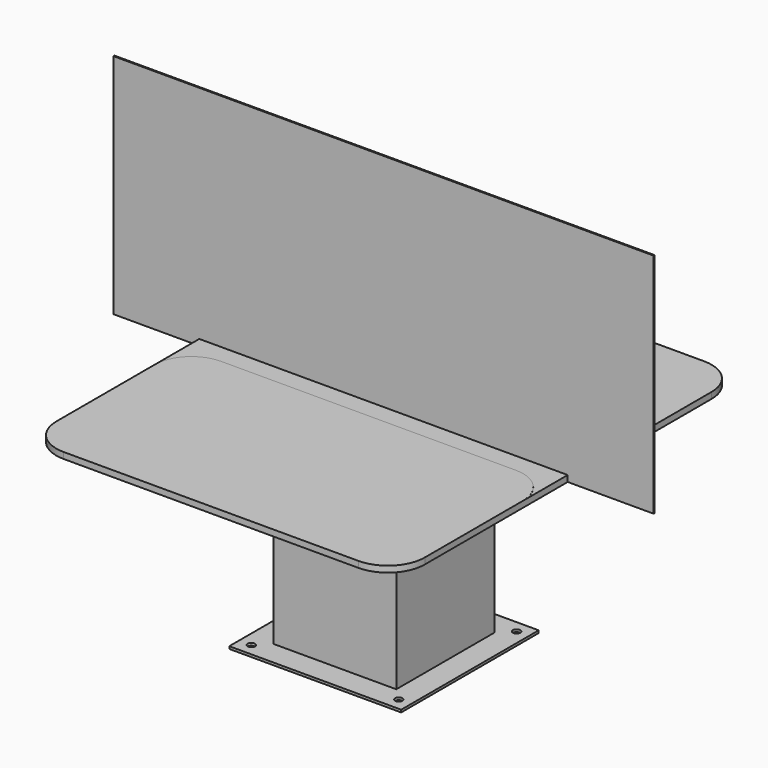
from build123d import *

# Parameters (mm, degrees)
F0_R      = 1250
F1_DEPTH  = 25
F3_DEPTH  = 0.1
F4_W      = 500
F4_H      = 500
F4_W_2    = 490
F4_H_2    = 490
F5_DEPTH  = 800
F6_W      = 2200
F6_H      = 5
F7_DEPTH  = 900
F8_W      = 500
F8_H      = 500
F9_DEPTH  = 5
F10_W     = 700
F10_H     = 700
F10_R     = 15
F11_DEPTH = 10
F13_DEPTH = 30
F15_DEPTH = 30
F16_W     = 490
F16_H     = 490
F17_DEPTH = 25
F18_R     = 350
F20_DEPTH = 25
F21_W     = 350
F21_H     = 25
F22_DEPTH = 5


# Not quite as in the source:
# - a feature names something its author has since deleted; it is built from what else it names


with BuildPart() as f1:
    # F0 (on Top) → F1 (new body)
    with BuildSketch(Plane.XY):
        Circle(F0_R)
    extrude(amount=F1_DEPTH)

    # F2 (on face) → F3 (join)
    with BuildSketch(Plane.XY.offset(25)):
        with BuildLine():
            Line((-600, 80), (600, 80))
            ThreePointArc((600, 80), (706.066017178, 123.933982822), (750, 230))
            Line((750, 230), (750, 730))
            ThreePointArc((750, 730), (706.066017178, 836.066017178), (600, 880))
            Line((600, 880), (-600, 880))
            ThreePointArc((-600, 880), (-706.066017178, 836.066017178), (-750, 730))
            Line((-750, 730), (-750, 230))
            ThreePointArc((-750, 230), (-706.066017178, 123.933982822), (-600, 80))
        make_face()
        with BuildLine():
            ThreePointArc((-600, -80), (-706.066017178, -123.933982822), (-750, -230))
            Line((-750, -230), (-750, -730))
            ThreePointArc((-750, -730), (-706.066017178, -836.066017178), (-600, -880))
            Line((-600, -880), (600, -880))
            ThreePointArc((600, -880), (706.066017178, -836.066017178), (750, -730))
            Line((750, -730), (750, -230))
            ThreePointArc((750, -230), (706.066017178, -123.933982822), (600, -80))
            Line((600, -80), (-600, -80))
        make_face()
    extrude(amount=F3_DEPTH)

    # F12 (on face) → F13 (cut)
    with BuildSketch(Plane.XY.offset(25)):
        with BuildLine():
            ThreePointArc((835.2245207129, -930), (0, -1250), (-835.2245207129, -930))
            Line((-835.2245207129, -930), (-1254.9974999975, -930))
            Line((-1254.9974999975, -930), (-1254.9974999975, -1430))
            Line((-1254.9974999975, -1430), (1245.0025000025, -1430))
            Line((1245.0025000025, -1430), (1245.0025000025, -930))
            Line((1245.0025000025, -930), (835.2245207129, -930))
        make_face()
        with BuildLine():
            Line((-835.2245207129, 930), (835.2245207129, 930))
            ThreePointArc((835.2245207129, 930), (0, 1250), (-835.2245207129, 930))
        make_face()
        with BuildLine():
            Line((835.2245207129, -930), (-835.2245207129, -930))
            ThreePointArc((-835.2245207129, -930), (0, -1250), (835.2245207129, -930))
        make_face()
    extrude(amount=-F13_DEPTH, mode=Mode.SUBTRACT)

    # F14 (on face) → F15 (cut)
    with BuildSketch(Plane.XY.offset(25)):
        Polygon((835.2245207128, 930), (835.2245207128, -930), (1324.2889336484, -826), (1324.2889336484, 930), align=None)
        Polygon((-1324.2889336484, -826), (-835.2245207128, -930), (-835.2245207128, 930), (-1324.2889336484, 930), align=None)
    extrude(amount=-F15_DEPTH, mode=Mode.SUBTRACT)

    # F18
    f18_edges = [f1.edges().sort_by_distance(p)[0] for p in [
        (-835.224521, 930, 12.5),
        (-835.224521, -930, 12.5),
        (835.224521, -930, 12.5),
        (835.224521, 930, 12.5),
    ]]
    fillet(f18_edges, radius=F18_R)

    # F19 (on face) → F20 (cut)
    with BuildSketch(Plane.XY.offset(25)):
        with BuildLine():
            Line((-750, 230), (-750, 730))
            ThreePointArc((-750, 730), (-730.6905446057, 803.6205239771), (-677.7335793245, 858.2867516363))
            Line((-677.7335793245, 858.2867516363), (-665.502084486, 880))
            ThreePointArc((-665.502084486, 880), (-789.8531038437, 752.3410175776), (-835.2245207128, 580))
            Line((-835.2245207128, 580), (-835.2245207128, -580))
            ThreePointArc((-835.2245207128, -580), (-813.2271256953, -702.1240808553), (-750, -808.8972380092))
            Line((-750, -808.8972380092), (-750, -730))
            Line((-750, -730), (-750, -230))
            Line((-750, -230), (-750, 230))
        make_face()
        with BuildLine():
            Line((-665.502084486, 880), (-677.7335793245, 858.2867516363))
            ThreePointArc((-677.7335793245, 858.2867516363), (-640.3545985889, 874.4697420664), (-600, 880))
            Line((-600, 880), (-665.502084486, 880))
        make_face()
        with BuildLine():
            ThreePointArc((-485.2245207128, 930), (-578.7659553822, 917.2684390808), (-665.502084486, 880))
            Line((-665.502084486, 880), (-600, 880))
            Line((-600, 880), (600, 880))
            Line((600, 880), (665.502084486, 880))
            ThreePointArc((665.502084486, 880), (578.7659553822, 917.2684390808), (485.2245207128, 930))
            Line((485.2245207128, 930), (-485.2245207128, 930))
        make_face()
        with BuildLine():
            ThreePointArc((-600, -880), (-706.066017178, -836.066017178), (-750, -730))
            Line((-750, -730), (-750, -808.8972380092))
            ThreePointArc((-750, -808.8972380092), (-710.5730362948, -847.8022526511), (-665.5020844861, -880))
            Line((-665.5020844861, -880), (-600, -880))
        make_face()
        with BuildLine():
            Line((665.502084486, 880), (600, 880))
            ThreePointArc((600, 880), (645.3424208849, 872.9827432535), (686.4424496518, 852.5875315772))
            Line((686.4424496518, 852.5875315772), (665.502084486, 880))
        make_face()
        with BuildLine():
            Line((600, -880), (-600, -880))
            Line((-600, -880), (-665.5020844861, -880))
            ThreePointArc((-665.5020844861, -880), (-578.7659553822, -917.2684390808), (-485.2245207128, -930))
            Line((-485.2245207128, -930), (485.2245207128, -930))
            ThreePointArc((485.2245207128, -930), (578.7659553822, -917.2684390808), (665.5020844861, -880))
            Line((665.5020844861, -880), (600, -880))
        make_face()
        with BuildLine():
            Line((750, 730), (750, 230))
            Line((750, 230), (750, -230))
            Line((750, -230), (750, -730))
            Line((750, -730), (750, -808.8972380092))
            ThreePointArc((750, -808.8972380092), (813.2271256953, -702.1240808553), (835.2245207128, -580))
            Line((835.2245207128, -580), (835.2245207128, 580))
            ThreePointArc((835.2245207128, 580), (789.8531038437, 752.3410175776), (665.502084486, 880))
            Line((665.502084486, 880), (686.4424496518, 852.5875315772))
            ThreePointArc((686.4424496518, 852.5875315772), (719.2000530228, 821.0568358739), (741.0058450449, 781.1600592569))
            Line((741.0058450449, 781.1600592569), (750, 769.3860530853))
            Line((750, 769.3860530853), (750, 730))
        make_face()
        with BuildLine():
            ThreePointArc((750, -730), (706.066017178, -836.066017178), (600, -880))
            Line((600, -880), (665.5020844861, -880))
            ThreePointArc((665.5020844861, -880), (710.5730362948, -847.8022526511), (750, -808.8972380092))
            Line((750, -808.8972380092), (750, -730))
        make_face()
        with BuildLine():
            ThreePointArc((741.0058450449, 781.1600592569), (747.7343507055, 755.9723241476), (750, 730))
            Line((750, 730), (750, 769.3860530853))
            Line((750, 769.3860530853), (741.0058450449, 781.1600592569))
        make_face()
    extrude(amount=-F20_DEPTH, mode=Mode.SUBTRACT)


with BuildPart() as f5:
    # F4 (on face) → F5 (new body)
    with BuildSketch(Plane(origin=(0, 0, 0), x_dir=(1, 0, 0), z_dir=(0, 0, -1))):
        Rectangle(F4_W, F4_H)
        Rectangle(F4_W_2, F4_H_2, mode=Mode.SUBTRACT)
    extrude(amount=F5_DEPTH)

    # F8 (on face) → F9 (join)
    with BuildSketch(Plane(origin=(0, 0, -800), x_dir=(1, 0, 0), z_dir=(0, 0, -1))):
        Rectangle(F8_W, F8_H)
    extrude(amount=F9_DEPTH)

    # F10 (on face) → F11 (join)
    with BuildSketch(Plane(origin=(0, 0, -805), x_dir=(1, 0, 0), z_dir=(0, 0, -1))):
        Rectangle(F10_W, F10_H)
        with Locations((-300, -300)):
            Circle(F10_R, mode=Mode.SUBTRACT)
        with Locations((300, -300)):
            Circle(F10_R, mode=Mode.SUBTRACT)
        with Locations((-300, 300)):
            Circle(F10_R, mode=Mode.SUBTRACT)
        with Locations((300, 300)):
            Circle(F10_R, mode=Mode.SUBTRACT)
    extrude(amount=F11_DEPTH)


with BuildPart() as f7:
    # F6 (on face) → F7 (new body)
    with BuildSketch(Plane.XY.offset(25)):
        Rectangle(F6_W, F6_H)
    extrude(amount=F7_DEPTH)

    # F21 (on face) → F22 (join)
    with BuildSketch(Plane.XZ.offset(2.5)):
        with Locations((-925, 12.5)):
            Rectangle(F21_W, F21_H)
        with Locations((925, 12.5)):
            Rectangle(F21_W, F21_H)
    extrude(amount=-F22_DEPTH)


with BuildPart() as f17:
    # F16 (on face) → F17 (new body)
    with BuildSketch(Plane.XY):
        Rectangle(F16_W, F16_H)
    extrude(amount=-F17_DEPTH)


solid = Compound([f1.part, f5.part, f7.part, f17.part])
